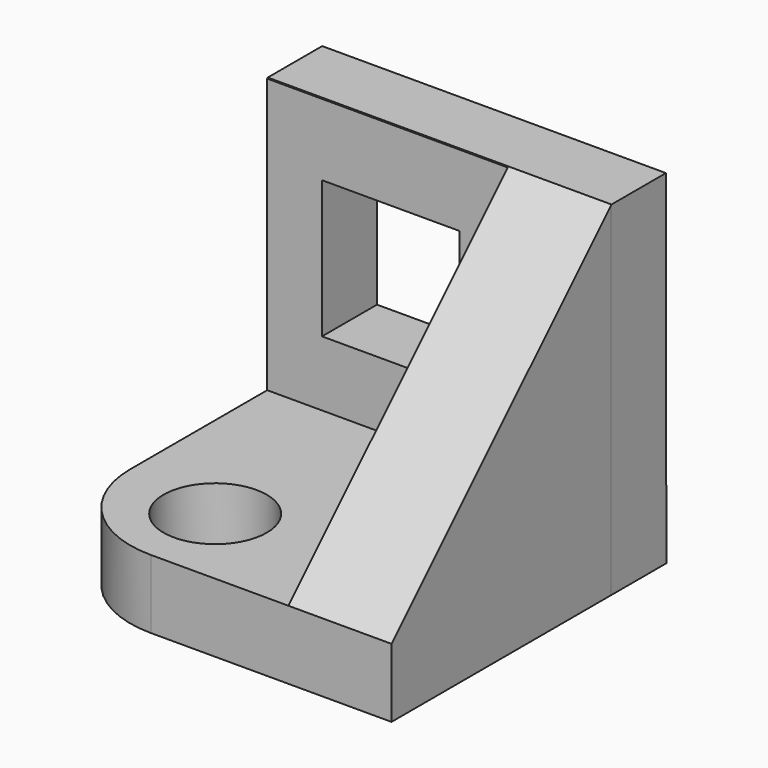
from build123d import *

# Parameters (mm, degrees)
F0_W        = 100
F0_H        = 100
F1_DEPTH    = 20
F2_R        = 30
F3_W        = 100
F3_H        = 20
F4_DEPTH    = 100
F5_W        = 30
F5_H        = 79.7933057844
F6_DEPTH    = 80
F7_T1_DEPTH = 441.4692780745
F8_R        = 15
F9_DEPTH    = 61.3
F10_W       = 40
F10_H       = 40
F11_DEPTH   = 41.8


# Not quite as in the source:
# - a fillet or chamfer that OpenCascade refuses, or shapes differently, is made with other operations: its cross-section is extruded or revolved along the edge and cut away or added


with BuildPart() as f1:
    # F0 (on Top) → F1 (new body)
    with BuildSketch(Plane.XY):
        Rectangle(F0_W, F0_H)
    extrude(amount=F1_DEPTH)

    # F2
    f2_edges = [f1.edges().sort_by_distance(p)[0] for p in [
        (-50, -50, 10),
    ]]
    fillet(f2_edges, radius=F2_R)

    # F3 (on Top) → F4 (join)
    with BuildSketch(Plane.XY):
        with Locations((4.657e-07, 39.7933057844)):
            Rectangle(F3_W, F3_H)
    extrude(amount=F4_DEPTH)

    # F5 (on face) → F6 (join)
    with BuildSketch(Plane.XY.offset(20)):
        with Locations((35, -10.1033471078)):
            Rectangle(F5_W, F5_H)
    extrude(amount=F6_DEPTH)

    # F7: chamfer of 80 on 1 edges, made by hand

    # F7_s2 → F7_t1 (cut)
    with BuildSketch(Plane.YZ.offset(-185.7346390373)):
        Polygon((-50, 20), (30, 100), (-50, 100), align=None)
    extrude(amount=F7_T1_DEPTH, mode=Mode.SUBTRACT)

    # F8 (on face) → F9 (cut)
    with BuildSketch(Plane.XY.offset(20)):
        with Locations((-21.275044793, -25.0325359563)):
            Circle(F8_R)
    extrude(amount=-F9_DEPTH, mode=Mode.SUBTRACT)

    # F10 (on face) → F11 (cut)
    with BuildSketch(Plane.XZ.offset(-29.7933057844)):
        with Locations((-14.0485025477, 58.9696498009)):
            Rectangle(F10_W, F10_H)
    extrude(amount=-F11_DEPTH, mode=Mode.SUBTRACT)


solid = f1.part
